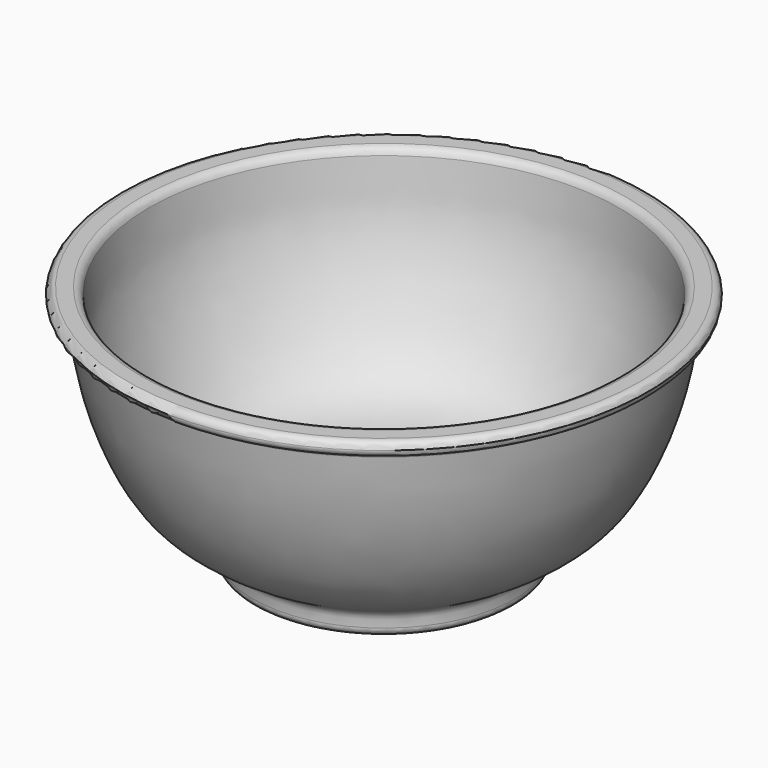
from build123d import *

# Parameters (mm, degrees)
F2_R           = 5.08
F5_D           = 4.4958
F5_CSINK_D     = 9.1186
F5_CSINK_ANGLE = 82
F6_R           = 3.25119


# Not quite as in the source:
# - a fillet or chamfer that OpenCascade refuses, or shapes differently, is made with other operations: its cross-section is extruded or revolved along the edge and cut away or added
# - a fillet or chamfer is up to 0.001 mm smaller than in the source, because OpenCascade refuses the exact size


with BuildPart() as f1:
    # F0 (on Front) → F1 (revolve)
    with BuildSketch(Plane.XZ):
        with BuildLine():
            Line((27.6298361897, -53.374024616), (46.6798361897, -53.374024616))
            Line((46.6798361897, -53.374024616), (46.6798361897, -37.9265157998))
            Line((46.6798361897, -37.9265157998), (27.6298361897, -37.9265157998))
            Line((27.6298361897, -37.9265157998), (27.6298361897, -25.2265157998))
            add(Edge.make_bspline(
                [(27.6298361897, -25.2265157998), (15.5749955494, -23.8777277254), (-2.3080647277, -19.248229525), (-21.5530079978, -2.8040698611), (-40.7052200015, 29.9060837396), (-53.2083366158, 69.0902566771), (-52.9778326059, 87.6604708421), (-54.9201638103, 105.375975384)],
                knots=[0, 0, 0, 0, 0.1906623549, 0.3587137849, 0.5714414191, 0.7860853721, 1, 1, 1, 1], degree=3))
            Line((-54.9201638103, 105.375975384), (-73.9701638103, 105.375975384))
            Line((-73.9701638103, 105.375975384), (-73.9701638103, 95.723975384))
            Line((-73.9701638103, 95.723975384), (-63.8101638103, 95.723975384))
            add(Edge.make_bspline(
                [(14.9298361897, -56.625224616), (15.4431777214, -53.374024616), (17.5886526762, -41.0990979254), (1.8258084828, -34.8824386954), (-25.1203339264, -15.923637622), (-39.50662959, 6.260147279), (-50.3811697961, 31.4707791655), (-58.2310879585, 58.1970989972), (-61.9810285963, 80.006964744), (-63.8101638103, 95.723975384)],
                knots=[0, 0, 0, 0, 0.1033040781, 0.2136177267, 0.377379662, 0.5255354297, 0.6733913097, 0.8214071996, 1, 1, 1, 1], degree=3))
            Line((14.9298361897, -56.625224616), (27.6298361897, -56.625224616))
            Line((27.6298361897, -56.625224616), (27.6298361897, -53.374024616))
        make_face()
    revolve(axis=Axis((103.8298361897, 0, 25.5734842002), (0, 0, -1)))

    # F2
    f2_edges = [f1.edges().sort_by_distance(p)[0] for p in [
        (281.629836, 0, 95.723975),
        (262.579836, 0, 105.375975),
        (192.729836, 0, -56.625225),
        (271.469836, 0, 95.723975),
    ]]
    fillet(f2_edges, radius=F2_R)

    # F3: fillet of radius 5.08 on 1 edges, made by hand

    # F3_s1 → F3_t2 (revolve, cut)
    with BuildSketch(Plane.XZ):
        with BuildLine():
            ThreePointArc((-73.9701638103, 100.803975384), (-72.3233952275, 104.0634042154), (-68.9156276298, 105.375975384))
            Line((-68.9156276298, 105.375975384), (-73.9701638103, 105.375975384))
            Line((-73.9701638103, 105.375975384), (-73.9701638103, 100.803975384))
        make_face()
    revolve(axis=Axis((103.8298361897, 0, 105.375975384), (0, 0, -1)), mode=Mode.SUBTRACT)

    # F5 (through all)
    with Locations(Plane(origin=(0, 0, -53.374024616), x_dir=(1, 0, 0), z_dir=(0, 0, -1))):
        with Locations((103.8298361897, 0), (137.1673361897, 57.7422437973), (137.1673361897, -57.7422437973), (37.1548361897, 0)):
            CounterSinkHole(F5_D / 2, F5_CSINK_D / 2, counter_sink_angle=F5_CSINK_ANGLE)

    # F6 (radius 3.2512 in the source; OpenCascade refuses exactly that, so slightly less here)
    f6_edges = [f1.edges().sort_by_distance(p)[0] for p in [
        (180.029836, 0, -56.625225),
    ]]
    fillet(f6_edges, radius=F6_R)


solid = f1.part
